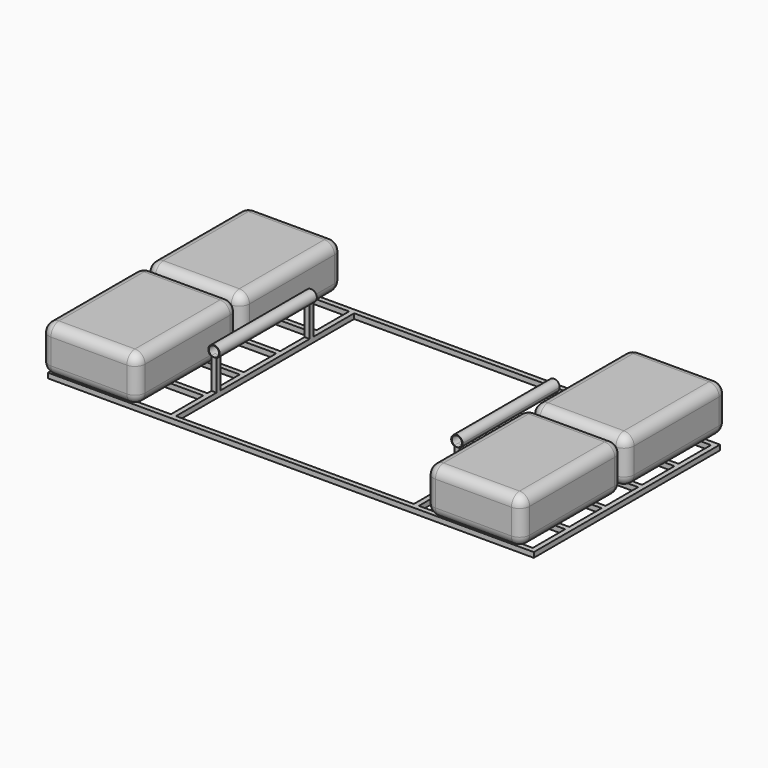
from build123d import *
from build123d import SkipClean  # not in build123d's __all__

# Parameters (mm, degrees)
F0_W     = 285.75
F0_H     = 12.7
F1_DEPTH = 12.7
F2_W     = 12.7
F2_H     = 12.7
F3_DEPTH = 88.9
F4_R     = 12.7
F5_DEPTH = 304.8
F4_R_2   = 14.2875
F6_DEPTH = 304.8
F8_W     = 241.3
F8_H     = 317.5
F9_DEPTH = 114.3
F10_R    = 25.4
F10_2_R  = 25.4
F10_3_R  = 25.4
F10_4_R  = 25.4


# Not quite as in the source:
# - a feature names something its author has since deleted; it is built from what else it names


with BuildPart() as f1:
    # F0 (on Top) → F1 (new body)
    with BuildSketch(Plane.XY):
        Polygon((609.6, 292.1), (0, 292.1), (-609.6, 292.1), (-609.6, 279.4), (-596.9, 279.4), (-311.15, 279.4), (-298.45, 279.4), (0, 279.4), (298.45, 279.4), (311.15, 279.4), (596.9, 279.4), (609.6, 279.4), align=None)
        Polygon((-596.9, 279.4), (-609.6, 279.4), (-609.6, -279.4), (-596.9, -279.4), (-596.9, -177.8), (-596.9, -165.1), (-596.9, -63.5), (-596.9, -50.8), (-596.9, 50.8), (-596.9, 63.5), (-596.9, 165.1), (-596.9, 177.8), align=None)
        Polygon((609.6, -279.4), (609.6, 279.4), (596.9, 279.4), (596.9, 177.8), (596.9, 165.1), (596.9, 63.5), (596.9, 50.8), (596.9, -50.8), (596.9, -63.5), (596.9, -165.1), (596.9, -177.8), (596.9, -279.4), align=None)
        Polygon((-596.9, -279.4), (-609.6, -279.4), (-609.6, -292.1), (0, -292.1), (609.6, -292.1), (609.6, -279.4), (596.9, -279.4), (311.15, -279.4), (298.45, -279.4), (0, -279.4), (-298.45, -279.4), (-311.15, -279.4), align=None)
        with Locations((-454.025, 171.45)):
            Rectangle(F0_W, F0_H)
        with Locations((-454.025, 57.15)):
            Rectangle(F0_W, F0_H)
        Polygon((-298.45, 279.4), (-311.15, 279.4), (-311.15, 177.8), (-311.15, 165.1), (-311.15, 63.5), (-311.15, 50.8), (-311.15, -50.8), (-311.15, -63.5), (-311.15, -165.1), (-311.15, -177.8), (-311.15, -279.4), (-298.45, -279.4), align=None)
        with Locations((-454.025, -57.15)):
            Rectangle(F0_W, F0_H)
        with Locations((-454.025, -171.45)):
            Rectangle(F0_W, F0_H)
        Polygon((311.15, 177.8), (311.15, 279.4), (298.45, 279.4), (298.45, -279.4), (311.15, -279.4), (311.15, -177.8), (311.15, -165.1), (311.15, -63.5), (311.15, -50.8), (311.15, 50.8), (311.15, 63.5), (311.15, 165.1), align=None)
        with Locations((454.025, 171.45)):
            Rectangle(F0_W, F0_H)
        with Locations((454.025, 57.15)):
            Rectangle(F0_W, F0_H)
        with Locations((454.025, -57.15)):
            Rectangle(F0_W, F0_H)
        with Locations((454.025, -171.45)):
            Rectangle(F0_W, F0_H)
    extrude(amount=F1_DEPTH)

    # F2 (on face) → F3 (join)
    with BuildSketch(Plane.XY.offset(12.7)):
        with Locations((-304.8, 146.05)):
            Rectangle(F2_W, F2_H)
        with Locations((-304.8, -146.05)):
            Rectangle(F2_W, F2_H)
        with Locations((304.8, -146.05)):
            Rectangle(F2_W, F2_H)
        with Locations((304.8, 146.05)):
            Rectangle(F2_W, F2_H)
    extrude(amount=F3_DEPTH)

    # F4 (on face) → F5 (cut, through all)
    with BuildSketch(Plane.XZ.offset(152.4)):
        with BuildLine():
            Line((298.45, 101.6), (298.45, 90.6014773719))
            ThreePointArc((298.45, 90.6014773719), (304.8, 88.9), (311.15, 90.6014773719))
            Line((311.15, 90.6014773719), (311.15, 101.6))
            Line((311.15, 101.6), (298.45, 101.6))
        make_face()
        with Locations((-304.8, 101.6)):
            Circle(F4_R)
    extrude(amount=-F5_DEPTH, mode=Mode.SUBTRACT)

    # F4 (on face) → F6 (join, through all)
    with BuildSketch(Plane.XZ.offset(152.4)):
        with BuildLine():
            Line((298.45, 90.6014773719), (298.45, 88.8011658246))
            ThreePointArc((298.45, 88.8011658246), (304.8, 87.3125), (311.15, 88.8011658246))
            Line((311.15, 88.8011658246), (311.15, 90.6014773719))
            ThreePointArc((311.15, 90.6014773719), (304.8, 88.9), (298.45, 90.6014773719))
        make_face()
        with Locations((-304.8, 101.6)):
            Circle(F4_R_2)
        with Locations((-304.8, 101.6)):
            Circle(F4_R, mode=Mode.SUBTRACT)
        with BuildLine():
            ThreePointArc((311.15, 88.8011658246), (316.9420402167, 94.0698263217), (319.0875, 101.6))
            ThreePointArc((319.0875, 101.6), (297.2698263217, 113.7420402167), (298.45, 88.8011658246))
            Line((298.45, 88.8011658246), (298.45, 90.6014773719))
            ThreePointArc((298.45, 90.6014773719), (298.45, 112.5985226281), (317.5, 101.6))
            ThreePointArc((317.5, 101.6), (315.7985226281, 95.25), (311.15, 90.6014773719))
            Line((311.15, 90.6014773719), (311.15, 88.8011658246))
        make_face()
    with SkipClean():  # cleaning this boolean's faces spoils the solid; the shape is the same uncleaned
        extrude(amount=-F6_DEPTH)


with BuildPart() as f9:
    # F8 (on offset) → F9 (new body)
    with BuildSketch(Plane.XY.offset(25)):
        with Locations((482.6, 163.75)):
            Rectangle(F8_W, F8_H)
    extrude(amount=F9_DEPTH)

    # F10#4
    f10_4_edges = [f9.edges().sort_by_distance(p)[0] for p in [
        (603.25, 163.75, 139.3),
        (482.6, 322.5, 139.3),
        (361.95, 163.75, 139.3),
        (482.6, 5, 139.3),
        (361.95, 322.5, 82.15),
        (361.95, 5, 82.15),
        (361.95, 163.75, 25),
        (603.25, 163.75, 25),
        (482.6, 322.5, 25),
        (482.6, 5, 25),
        (603.25, 5, 82.15),
        (603.25, 322.5, 82.15),
    ]]
    fillet(f10_4_edges, radius=F10_4_R)


with BuildPart() as f9b:
    # F8 (on offset) → F9, piece 2 (new body)
    with BuildSketch(Plane.XY.offset(25)):
        with Locations((482.6, -163.75)):
            Rectangle(F8_W, F8_H)
    extrude(amount=F9_DEPTH)

    # F10#3
    f10_3_edges = [f9b.edges().sort_by_distance(p)[0] for p in [
        (482.6, -322.5, 139.3),
        (603.25, -163.75, 139.3),
        (482.6, -5, 139.3),
        (361.95, -163.75, 139.3),
        (361.95, -5, 82.15),
        (361.95, -322.5, 82.15),
        (361.95, -163.75, 25),
        (482.6, -322.5, 25),
        (603.25, -163.75, 25),
        (482.6, -5, 25),
        (603.25, -322.5, 82.15),
        (603.25, -5, 82.15),
    ]]
    fillet(f10_3_edges, radius=F10_3_R)


with BuildPart() as f9c:
    # F8 (on offset) → F9, piece 3 (new body)
    with BuildSketch(Plane.XY.offset(25)):
        with Locations((-482.6, 163.75)):
            Rectangle(F8_W, F8_H)
    extrude(amount=F9_DEPTH)

    # F10
    f10_edges = [f9c.edges().sort_by_distance(p)[0] for p in [
        (-603.25, 163.75, 139.3),
        (-482.6, 5, 139.3),
        (-361.95, 163.75, 139.3),
        (-482.6, 322.5, 139.3),
        (-603.25, 322.5, 82.15),
        (-603.25, 5, 82.15),
        (-603.25, 163.75, 25),
        (-482.6, 5, 25),
        (-361.95, 163.75, 25),
        (-482.6, 322.5, 25),
        (-361.95, 5, 82.15),
        (-361.95, 322.5, 82.15),
    ]]
    fillet(f10_edges, radius=F10_R)


with BuildPart() as f9d:
    # F8 (on offset) → F9, piece 4 (new body)
    with BuildSketch(Plane.XY.offset(25)):
        with Locations((-482.6, -163.75)):
            Rectangle(F8_W, F8_H)
    extrude(amount=F9_DEPTH)

    # F10#2
    f10_2_edges = [f9d.edges().sort_by_distance(p)[0] for p in [
        (-482.6, -322.5, 139.3),
        (-361.95, -163.75, 139.3),
        (-482.6, -5, 139.3),
        (-603.25, -163.75, 139.3),
        (-603.25, -5, 82.15),
        (-603.25, -322.5, 82.15),
        (-603.25, -163.75, 25),
        (-482.6, -322.5, 25),
        (-361.95, -163.75, 25),
        (-482.6, -5, 25),
        (-361.95, -322.5, 82.15),
        (-361.95, -5, 82.15),
    ]]
    fillet(f10_2_edges, radius=F10_2_R)


solid = Compound([f1.part, f9.part, f9b.part, f9c.part, f9d.part])
